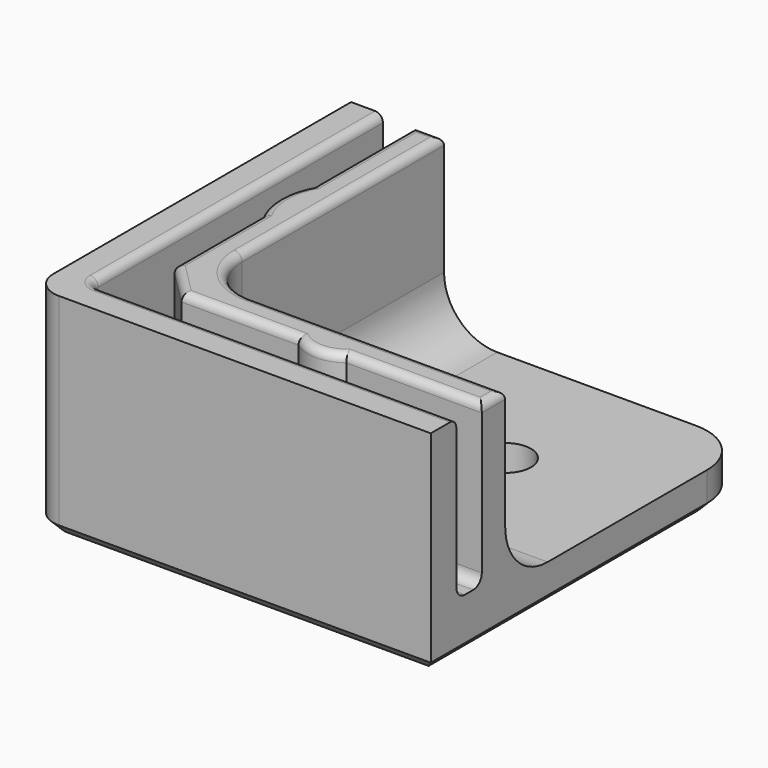
from build123d import *

# Parameters (mm, degrees)
F0_W          = 38.1
F0_H          = 38.1
F1_DEPTH      = 20.32
F2_W          = 29.21
F2_H          = 29.21
F3_DEPTH      = 16.51
F5_DEPTH      = 15.24
F6_T1_DEPTH   = 29.21
F7_R          = 5.08
F8_R          = 5.08
F9_R          = 2.54
F10_R         = 2.413
F11_DEPTH     = 20.321
F13_DEPTH     = 15.24
F14_T1_DEPTH  = 14.224
F14_T3_DEPTH  = 34.036
F14_T5_DEPTH  = 34.036
F14_T7_DEPTH  = 19.05
F14_T9_DEPTH  = 18.3199171099
F14_S13_W     = 1.03632
F14_S13_H     = 1.03632
F14_T14_DEPTH = 1.03632
F14_T20_DEPTH = 16.861733183
F14_T26_DEPTH = 22.6379171099
F14_T31_DEPTH = 23.368
F14_T36_ANGLE = 257.1357278548
F14_T42_DEPTH = 16.861733183
F14_T46_DEPTH = 23.368
F14_T53_DEPTH = 16.861733183
F14_T57_DEPTH = 22.6379171099
F15_SIZE      = 1.016
F16_R         = 0.762


# Not quite as in the source:
# - a fillet or chamfer that OpenCascade refuses, or shapes differently, is made with other operations: its cross-section is extruded or revolved along the edge and cut away or added


with BuildPart() as f1:
    # F0 (on Top) → F1 (new body)
    with BuildSketch(Plane.XY):
        with Locations((19.05, 19.05)):
            Rectangle(F0_W, F0_H)
    extrude(amount=F1_DEPTH)

    # F2 (on face) → F3 (cut)
    with BuildSketch(Plane.XY.offset(20.32)):
        with Locations((23.495, 23.495)):
            Rectangle(F2_W, F2_H)
    extrude(amount=-F3_DEPTH, mode=Mode.SUBTRACT)

    # F4 (on face) → F5 (cut)
    with BuildSketch(Plane.XY.offset(20.32)):
        Polygon((6.096, 38.1), (3.048, 38.1), (3.048, 3.048), (38.1, 3.048), (38.1, 6.096), (9.398, 6.096), (6.096, 6.096), (6.096, 9.398), align=None)
        Polygon((9.398, 6.096), (6.096, 9.398), (6.096, 6.096), align=None)
    extrude(amount=-F5_DEPTH, mode=Mode.SUBTRACT)

    # F6: fillet of radius 5.08 on 1 edges, made by hand

    # F6_s2 → F6_t1 (cut)
    with BuildSketch(Plane.XY.offset(-12.7)):
        with BuildLine():
            ThreePointArc((33.02, 38.1), (36.6121024484, 36.6121024484), (38.1, 33.02))
            Line((38.1, 33.02), (38.1, 38.1))
            Line((38.1, 38.1), (33.02, 38.1))
        make_face()
    extrude(amount=F6_T1_DEPTH, mode=Mode.SUBTRACT)

    # F7
    f7_edges = [f1.edges().sort_by_distance(p)[0] for p in [
        (8.89, 8.89, 12.065),
    ]]
    fillet(f7_edges, radius=F7_R)

    # F8
    f8_edges = [f1.edges().sort_by_distance(p)[0] for p in [
        (26.035, 8.89, 3.81),
        (10.377898, 10.377898, 3.81),
        (8.89, 26.035, 3.81),
    ]]
    fillet(f8_edges, radius=F8_R)

    # F9
    f9_edges = [f1.edges().sort_by_distance(p)[0] for p in [
        (0, 0, 10.16),
    ]]
    fillet(f9_edges, radius=F9_R)

    # F10 (on face) → F11 (cut, through all)
    with BuildSketch(Plane(origin=(0, 0, 0), x_dir=(1, 0, 0), z_dir=(0, 0, -1))):
        with Locations((25.144717139, -25.144717139)):
            Circle(F10_R)
    extrude(amount=-F11_DEPTH, mode=Mode.SUBTRACT)

    # F12 (on face) → F13 (join, through all)
    with BuildSketch(Plane.XY.offset(20.32)):
        with BuildLine():
            Line((25.146, 6.096), (20.574, 6.096))
            ThreePointArc((20.574, 6.096), (22.86, 5.334), (25.146, 6.096))
        make_face()
        with BuildLine():
            Line((6.096, 19.8439171099), (6.096, 25.8760828901))
            ThreePointArc((6.096, 25.8760828901), (5.334, 22.86), (6.096, 19.8439171099))
        make_face()
    extrude(amount=-F13_DEPTH)

    # F14: fillet of radius 1.016 on 9 edges, made by hand

    # F14_s2 → F14_t1 (join)
    with BuildSketch(Plane.XY.offset(6.096)):
        with BuildLine():
            ThreePointArc((4.064, 3.048), (3.3455795103, 3.3455795103), (3.048, 4.064))
            Line((3.048, 4.064), (3.02768, 4.064))
            Line((3.02768, 4.064), (3.02768, 3.02768))
            Line((3.02768, 3.02768), (4.064, 3.02768))
            Line((4.064, 3.02768), (4.064, 3.048))
        make_face()
    extrude(amount=F14_T1_DEPTH)

    # F14_s4 → F14_t3 (join)
    with BuildSketch(Plane.YZ.offset(4.064)):
        with BuildLine():
            ThreePointArc((4.064, 5.08), (3.3455795103, 5.3775795103), (3.048, 6.096))
            Line((3.048, 6.096), (3.02768, 6.096))
            Line((3.02768, 6.096), (3.02768, 5.05968))
            Line((3.02768, 5.05968), (4.064, 5.05968))
            Line((4.064, 5.05968), (4.064, 5.08))
        make_face()
    extrude(amount=F14_T3_DEPTH)

    # F14_s6 → F14_t5 (join)
    with BuildSketch(Plane.XZ.offset(-38.1)):
        with BuildLine():
            ThreePointArc((4.064, 5.08), (3.3455795103, 5.3775795103), (3.048, 6.096))
            Line((3.048, 6.096), (3.02768, 6.096))
            Line((3.02768, 6.096), (3.02768, 5.05968))
            Line((3.02768, 5.05968), (4.064, 5.05968))
            Line((4.064, 5.05968), (4.064, 5.08))
        make_face()
    extrude(amount=F14_T5_DEPTH)

    # F14_s8 → F14_t7 (join)
    with BuildSketch(Plane.YZ.offset(19.05)):
        with BuildLine():
            ThreePointArc((6.096, 6.096), (5.7984204897, 5.3775795103), (5.08, 5.08))
            Line((5.08, 5.08), (5.08, 5.05968))
            Line((5.08, 5.05968), (6.11632, 5.05968))
            Line((6.11632, 5.05968), (6.11632, 6.096))
            Line((6.11632, 6.096), (6.096, 6.096))
        make_face()
    extrude(amount=F14_T7_DEPTH)

    # F14_s10 → F14_t9 (join)
    with BuildSketch(Plane.XZ.offset(-38.1)):
        with BuildLine():
            ThreePointArc((5.08, 5.08), (5.7984204897, 5.3775795103), (6.096, 6.096))
            Line((6.096, 6.096), (6.11632, 6.096))
            Line((6.11632, 6.096), (6.11632, 5.05968))
            Line((6.11632, 5.05968), (5.08, 5.05968))
            Line((5.08, 5.05968), (5.08, 5.08))
        make_face()
    extrude(amount=F14_T9_DEPTH)


with BuildPart() as f14_tool12:
    # F14_s13 → F14_t14 (new body)
    with BuildSketch(Plane.YZ.offset(4.064)):
        with Locations((3.54584, 5.57784)):
            Rectangle(F14_S13_W, F14_S13_H)
    extrude(amount=-F14_T14_DEPTH)

    # F14_s15 → F14_t16 (revolve, cut)
    with BuildSketch(Plane(origin=(4.064, 4.064, 6.096), x_dir=(0, 0.7071067812, 0.7071067812), z_dir=(0, -0.7071067812, 0.7071067812))):
        with BuildLine():
            ThreePointArc((0, -1.016), (1.016, 0), (0, 1.016))
            Line((0, 1.016), (0, -1.016))
        make_face()
    revolve(axis=Axis((4.064, 4.064, 6.096), (-1, 0, 0)), mode=Mode.SUBTRACT)


with BuildPart() as f1_1:
    add(f1.part)

    # F14_t11: union F14_tool12
    add(f14_tool12.part)


with BuildPart() as f14_tool18:
    # F14_s19 → F14_t20 (new body)
    with BuildSketch(Plane(origin=(5.9615229381, -5.9615229381, 0), x_dir=(0, 0, 1), z_dir=(-0.7071067812, 0.7071067812, 0))):
        with BuildLine():
            ThreePointArc((5.08, 9.9399124677), (5.3775795103, 10.6583329574), (6.096, 10.9559124677))
            Line((6.096, 10.9559124677), (6.096, 10.9762324677))
            Line((6.096, 10.9762324677), (5.05968, 10.9762324677))
            Line((5.05968, 10.9762324677), (5.05968, 9.9399124677))
            Line((5.05968, 9.9399124677), (5.08, 9.9399124677))
        make_face()
    extrude(amount=F14_T20_DEPTH)

    split(bisect_by=Plane.YZ.offset(6.096), keep=Keep.TOP)

    split(bisect_by=Plane.XZ.offset(-6.096), keep=Keep.BOTTOM)


with BuildPart() as f1_2:
    add(f1_1.part)

    # F14_t17: union F14_tool18
    add(f14_tool18.part)


with BuildPart() as f14_tool24:
    # F14_s25 → F14_t26 (new body)
    with BuildSketch(Plane.XZ.offset(-3.302)):
        with BuildLine():
            ThreePointArc((5.08, 5.08), (5.7984204897, 5.3775795103), (6.096, 6.096))
            Line((6.096, 6.096), (6.11632, 6.096))
            Line((6.11632, 6.096), (6.11632, 5.05968))
            Line((6.11632, 5.05968), (5.08, 5.05968))
            Line((5.08, 5.05968), (5.08, 5.08))
        make_face()
    extrude(amount=-F14_T26_DEPTH)

    split(bisect_by=Plane(origin=(7.747, 7.747, 0), x_dir=(0, 0, 1), z_dir=(0.7071067812, 0.7071067812, 0)), keep=Keep.TOP)


with BuildPart() as f1_3:
    add(f1_2.part)

    # F14_t23: union F14_tool24
    add(f14_tool24.part)


with BuildPart() as f14_tool29:
    # F14_s30 → F14_t31 (new body)
    with BuildSketch(Plane.YZ.offset(26.67)):
        with BuildLine():
            ThreePointArc((5.08, 5.08), (5.7984204897, 5.3775795103), (6.096, 6.096))
            Line((6.096, 6.096), (6.11632, 6.096))
            Line((6.11632, 6.096), (6.11632, 5.05968))
            Line((6.11632, 5.05968), (5.08, 5.05968))
            Line((5.08, 5.05968), (5.08, 5.08))
        make_face()
    extrude(amount=-F14_T31_DEPTH)

    split(bisect_by=Plane(origin=(7.747, 7.747, 0), x_dir=(0, 0, 1), z_dir=(0.7071067812, 0.7071067812, 0)), keep=Keep.TOP)


with BuildPart() as f1_4:
    add(f1_3.part)

    # F14_t28: union F14_tool29
    add(f14_tool29.part)


with BuildPart() as f14_tool34:
    # F14_s35 → F14_t36 (revolve)
    with BuildSketch(Plane(origin=(13.3424429627, 16.7330298048, 0), x_dir=(0, 0, 1), z_dir=(0.6234411592, 0.7818702712, 0))):
        with BuildLine():
            ThreePointArc((5.08, 7.3468084408), (5.3775795103, 8.0652289305), (6.096, 8.3628084408))
            Line((6.096, 8.3628084408), (6.096, 8.3831284408))
            Line((6.096, 8.3831284408), (5.05968, 8.3831284408))
            Line((5.05968, 8.3831284408), (5.05968, 7.3468084408))
            Line((5.05968, 7.3468084408), (5.08, 7.3468084408))
        make_face()
    revolve(axis=Axis((22.86, 9.144, 5.08), (0, 0, 1)), revolution_arc=F14_T36_ANGLE)

    split(bisect_by=Plane.XZ.offset(-6.096), keep=Keep.TOP)


with BuildPart() as f1_5:
    add(f1_4.part)

    # F14_t33: union F14_tool34
    add(f14_tool34.part)


with BuildPart() as f14_tool40:
    # F14_s41 → F14_t42 (new body)
    with BuildSketch(Plane(origin=(5.9615229381, -5.9615229381, 0), x_dir=(0, 0, 1), z_dir=(-0.7071067812, 0.7071067812, 0))):
        with BuildLine():
            ThreePointArc((5.08, 9.9399124677), (5.3775795103, 10.6583329574), (6.096, 10.9559124677))
            Line((6.096, 10.9559124677), (6.096, 10.9762324677))
            Line((6.096, 10.9762324677), (5.05968, 10.9762324677))
            Line((5.05968, 10.9762324677), (5.05968, 9.9399124677))
            Line((5.05968, 9.9399124677), (5.08, 9.9399124677))
        make_face()
    extrude(amount=F14_T42_DEPTH)

    split(bisect_by=Plane.XZ.offset(-6.096), keep=Keep.TOP)


with BuildPart() as f14_tool44:
    # F14_s45 → F14_t46 (new body)
    with BuildSketch(Plane.YZ.offset(26.67)):
        with BuildLine():
            ThreePointArc((5.08, 5.08), (5.7984204897, 5.3775795103), (6.096, 6.096))
            Line((6.096, 6.096), (6.11632, 6.096))
            Line((6.11632, 6.096), (6.11632, 5.05968))
            Line((6.11632, 5.05968), (5.08, 5.05968))
            Line((5.08, 5.05968), (5.08, 5.08))
        make_face()
    extrude(amount=-F14_T46_DEPTH)

    split(bisect_by=Plane(origin=(7.747, 7.747, 0), x_dir=(0, 0, 1), z_dir=(-0.7071067812, -0.7071067812, 0)), keep=Keep.TOP)


with BuildPart() as f14_tool40_1:
    add(f14_tool40.part)

    # F14_t48: intersect F14_tool44
    add(f14_tool44.part, mode=Mode.INTERSECT)


with BuildPart() as f1_6:
    add(f1_5.part)

    # F14_t38: union F14_tool40
    add(f14_tool40_1.part)


with BuildPart() as f14_tool51:
    # F14_s52 → F14_t53 (new body)
    with BuildSketch(Plane(origin=(5.9615229381, -5.9615229381, 0), x_dir=(0, 0, 1), z_dir=(-0.7071067812, 0.7071067812, 0))):
        with BuildLine():
            ThreePointArc((5.08, 9.9399124677), (5.3775795103, 10.6583329574), (6.096, 10.9559124677))
            Line((6.096, 10.9559124677), (6.096, 10.9762324677))
            Line((6.096, 10.9762324677), (5.05968, 10.9762324677))
            Line((5.05968, 10.9762324677), (5.05968, 9.9399124677))
            Line((5.05968, 9.9399124677), (5.08, 9.9399124677))
        make_face()
    extrude(amount=F14_T53_DEPTH)

    split(bisect_by=Plane.YZ.offset(6.096), keep=Keep.BOTTOM)


with BuildPart() as f14_tool55:
    # F14_s56 → F14_t57 (new body)
    with BuildSketch(Plane.XZ.offset(-3.302)):
        with BuildLine():
            ThreePointArc((5.08, 5.08), (5.7984204897, 5.3775795103), (6.096, 6.096))
            Line((6.096, 6.096), (6.11632, 6.096))
            Line((6.11632, 6.096), (6.11632, 5.05968))
            Line((6.11632, 5.05968), (5.08, 5.05968))
            Line((5.08, 5.05968), (5.08, 5.08))
        make_face()
    extrude(amount=-F14_T57_DEPTH)

    split(bisect_by=Plane(origin=(7.747, 7.747, 0), x_dir=(0, 0, 1), z_dir=(-0.7071067812, -0.7071067812, 0)), keep=Keep.TOP)


with BuildPart() as f14_tool51_1:
    add(f14_tool51.part)

    # F14_t59: intersect F14_tool55
    add(f14_tool55.part, mode=Mode.INTERSECT)


with BuildPart() as f1_7:
    add(f1_6.part)

    # F14_t49: union F14_tool51
    add(f14_tool51_1.part)

    # F15
    f15_edges = [f1_7.edges().sort_by_distance(p)[0] for p in [
        (20.32, 0, 0),
        (16.51, 38.1, 0),
        (36.612102, 36.612102, 0),
        (0.743949, 0.743949, 0),
        (38.1, 16.51, 0),
        (0, 20.32, 0),
    ]]
    chamfer(f15_edges, length=F15_SIZE)

    # F16
    f16_edges = [f1_7.edges().sort_by_distance(p)[0] for p in [
        (3.048, 21.082, 20.32),
        (31.623, 6.096, 20.32),
        (22.86, 5.334, 20.32),
        (8.89, 26.035, 20.32),
        (7.493, 38.1, 20.32),
        (6.096, 31.988041, 20.32),
        (5.334, 22.86, 20.32),
        (6.096, 14.620959, 20.32),
        (7.747, 7.747, 20.32),
        (14.986, 6.096, 20.32),
        (38.1, 7.493, 20.32),
        (26.035, 8.89, 20.32),
        (10.377898, 10.377898, 20.32),
        (21.082, 3.048, 20.32),
        (3.34558, 3.34558, 20.32),
    ]]
    fillet(f16_edges, radius=F16_R)


solid = f1_7.part
